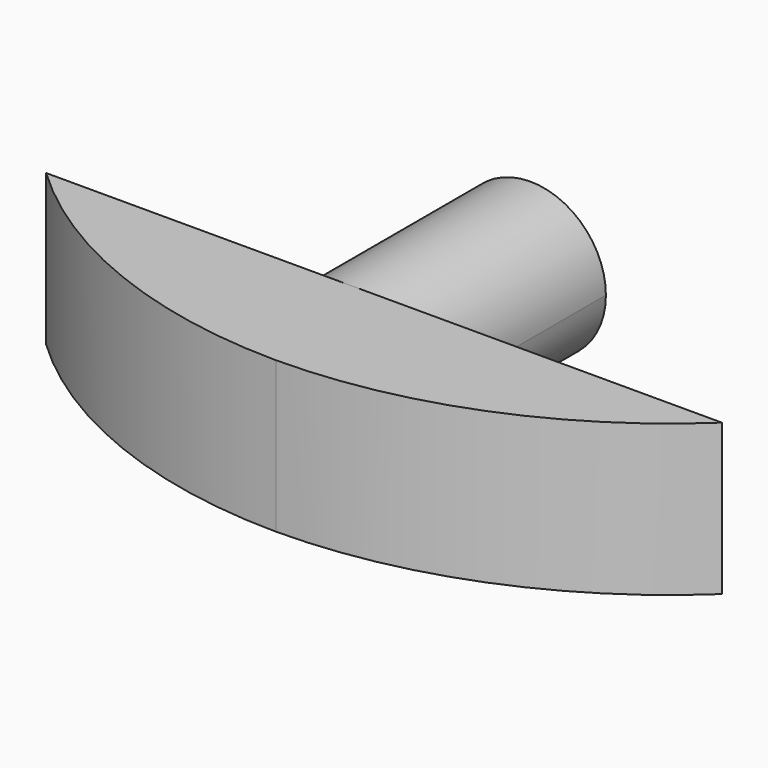
from build123d import *

# Parameters (mm, degrees)
F1_DEPTH    = 6
F2_DEPTH    = 10
F3_T1_DEPTH = 82.1983443527


# Not quite as in the source:
# - a fillet or chamfer that OpenCascade refuses, or shapes differently, is made with other operations: its cross-section is extruded or revolved along the edge and cut away or added


with BuildPart() as f1:
    # F0 (on Front) → F1 (new body)
    with BuildSketch(Plane.XZ):
        with BuildLine():
            Line((10.5583761781, 15.9778866861), (-19.4416238219, 15.9778866861))
            Line((-19.4416238219, 15.9778866861), (-19.4416238219, 9.2778866861))
            Line((-19.4416238219, 9.2778866861), (-6.2031285903, 9.2778866861))
            ThreePointArc((-6.2031285903, 9.2778866861), (-8.2160972802, 15.0771908879), (-2.5916238219, 12.6176644117))
            ThreePointArc((-2.5916238219, 12.6176644117), (-3.4820973456, 10.3431909533), (-5.6801190534, 9.2778866861))
            Line((-5.6801190534, 9.2778866861), (10.5583761781, 9.2778866861))
            Line((10.5583761781, 9.2778866861), (10.5583761781, 15.9778866861))
        make_face()
        with BuildLine():
            ThreePointArc((-2.5916238219, 12.6176644117), (-8.2160972802, 15.0771908879), (-6.2031285903, 9.2778866861))
            Line((-6.2031285903, 9.2778866861), (-5.6801190534, 9.2778866861))
            ThreePointArc((-5.6801190534, 9.2778866861), (-3.4820973456, 10.3431909533), (-2.5916238219, 12.6176644117))
        make_face()
    extrude(amount=F1_DEPTH)

    # F0 (on Front) → F2 (join)
    with BuildSketch(Plane.XZ):
        with BuildLine():
            ThreePointArc((-2.5916238219, 12.6176644117), (-8.2160972802, 15.0771908879), (-6.2031285903, 9.2778866861))
            Line((-6.2031285903, 9.2778866861), (-5.6801190534, 9.2778866861))
            ThreePointArc((-5.6801190534, 9.2778866861), (-3.4820973456, 10.3431909533), (-2.5916238219, 12.6176644117))
        make_face()
    extrude(amount=-F2_DEPTH)

    # F3: fillet of radius 22 on 2 edges, made by hand

    # F3_s2 → F3_t1 (cut)
    with BuildSketch(Plane.XY.offset(-28.4712854902)):
        with BuildLine():
            ThreePointArc((-19.4416238219, 0), (-12.4659933559, -4.4450483003), (-4.3419549513, -6))
            Line((-4.3419549513, -6), (-19.4416238219, -6))
            Line((-19.4416238219, -6), (-19.4416238219, 0))
        make_face()
        with BuildLine():
            ThreePointArc((10.5583761781, 0), (3.5827457122, -4.4450483003), (-4.5412926924, -6))
            Line((-4.5412926924, -6), (10.5583761781, -6))
            Line((10.5583761781, -6), (10.5583761781, 0))
        make_face()
    extrude(amount=F3_T1_DEPTH, mode=Mode.SUBTRACT)


solid = f1.part
